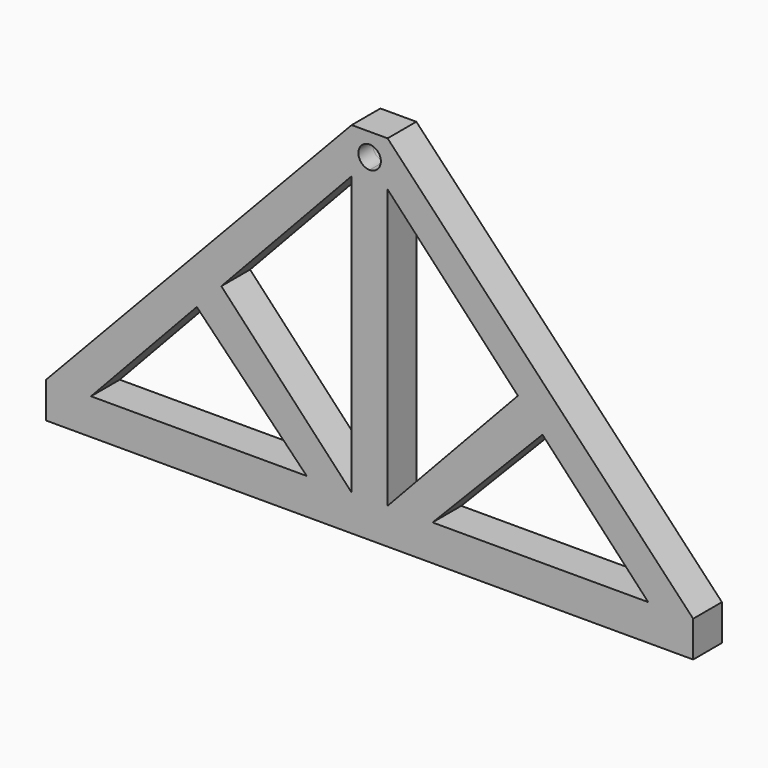
from build123d import *

# Parameters (mm, degrees)
F0_W     = 50.8
F0_H     = 101.6
F1_DEPTH = 50.8


with BuildPart() as f1:
    # F0 (on Front) → F1 (new body, symmetric)
    with BuildSketch(Plane.XZ):
        Polygon((-488.5087642836, 0), (-419.1, 74.1955756135), (-50.8, 467.8955756135), (-50.8, 594.8955756135), (-914.4, -319.5044243865), (-787.4, -319.5044243865), align=None)
        Polygon((-177.8, -319.5044243865), (-50.8, -319.5044243865), (-419.1, 74.1955756135), (-488.5087642836, 0), align=None)
        Polygon((-50.8, -421.1044243865), (-50.8, -319.5044243865), (-177.8, -319.5044243865), (-787.4, -319.5044243865), (-914.4, -319.5044243865), (-914.4, -421.1044243865), align=None)
        with BuildLine():
            Line((-50.8, -319.5044243865), (0, -319.5044243865))
            Line((0, -319.5044243865), (0, 499.6455756135))
            ThreePointArc((0, 499.6455756135), (-31.75, 531.3955756135), (0, 563.1455756135))
            Line((0, 563.1455756135), (0, 594.8955756135))
            Line((0, 594.8955756135), (-50.8, 594.8955756135))
            Line((-50.8, 594.8955756135), (-50.8, 467.8955756135))
            Line((-50.8, 467.8955756135), (-50.8, -319.5044243865))
        make_face()
        with BuildLine():
            Line((0, 499.6455756135), (0, -319.5044243865))
            Line((0, -319.5044243865), (50.8, -319.5044243865))
            Line((50.8, -319.5044243865), (50.8, 467.8955756135))
            Line((50.8, 467.8955756135), (50.8, 594.8955756135))
            Line((50.8, 594.8955756135), (0, 594.8955756135))
            Line((0, 594.8955756135), (0, 563.1455756135))
            ThreePointArc((0, 563.1455756135), (22.4506403027, 553.8462159162), (31.75, 531.3955756135))
            ThreePointArc((31.75, 531.3955756135), (22.4506403027, 508.9449353108), (0, 499.6455756135))
        make_face()
        with Locations((25.4, -370.3044243865)):
            Rectangle(F0_W, F0_H)
        with Locations((-25.4, -370.3044243865)):
            Rectangle(F0_W, F0_H)
        Polygon((177.8, -319.5044243865), (50.8, -319.5044243865), (50.8, -421.1044243865), (914.4, -421.1044243865), (914.4, -319.5044243865), (787.4, -319.5044243865), align=None)
        Polygon((50.8, 594.8955756135), (50.8, 467.8955756135), (419.1, 74.1955756135), (488.5087642836, 0), (787.4, -319.5044243865), (914.4, -319.5044243865), align=None)
        Polygon((419.1, 74.1955756135), (50.8, -319.5044243865), (177.8, -319.5044243865), (488.5087642836, 0), align=None)
    extrude(amount=F1_DEPTH, both=True)


solid = f1.part
